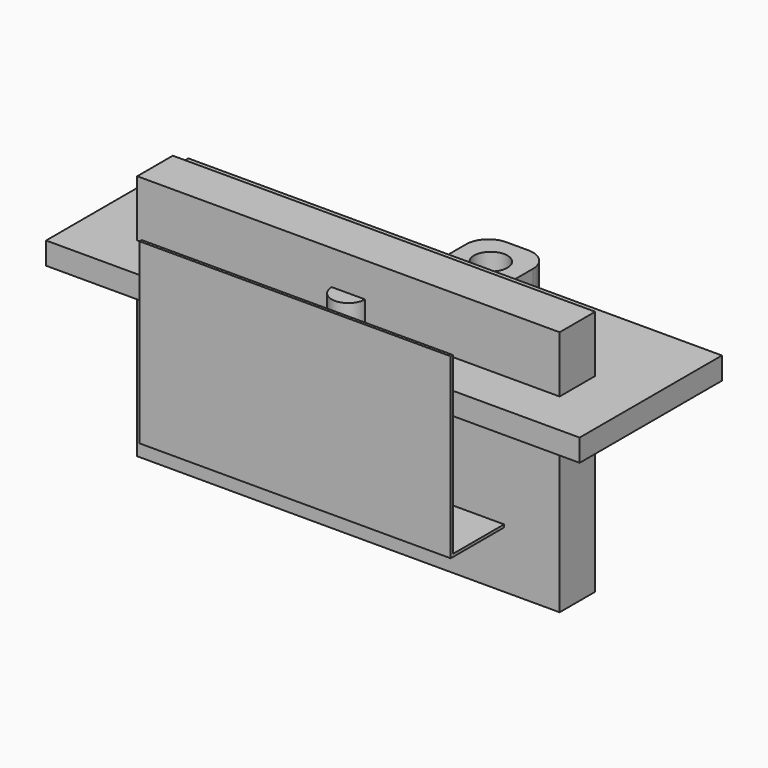
from build123d import *

# Parameters (mm, degrees)
F0_R           = 25.4
F1_DEPTH       = 50.8
F2_R           = 19.05
F3_DEPTH       = 50.8
F4_W           = 76.2
F4_H           = 254
F4_R           = 19.05
F5_DEPTH       = 50.8
F6_R           = 19.05
F7_DEPTH       = 50.8
F8_R           = 25.4
F9_R           = 38.1
F9_R_2         = 19.05
F10_DEPTH      = 50.8
F11_W          = 609.6
F11_H          = 203.2
F12_DEPTH      = 25.4
F13_R          = 19.05
F14_DEPTH      = 50.8
F15_W          = 482.6
F15_H          = 281.6996272628
F16_DEPTH      = 50.8
F17_R          = 25.4
F18_DEPTH      = 50.8
F20_DEPTH      = 177.8
F20_DEPTH_BACK = 177.8


with BuildPart() as f1:
    # F0 (on Top) → F1 (new body)
    with BuildSketch(Plane.XY):
        with BuildLine():
            ThreePointArc((-50.8, 0), (0, -50.8), (50.8, 0))
            ThreePointArc((50.8, 0), (0, 50.8), (-50.8, 0))
        make_face()
        Circle(F0_R, mode=Mode.SUBTRACT)
        with BuildLine():
            Line((50.8, -152.4), (50.8, 0))
            ThreePointArc((50.8, 0), (0, -50.8), (-50.8, 0))
            Line((-50.8, 0), (-50.8, -152.4))
            Line((-50.8, -152.4), (50.8, -152.4))
        make_face()
    extrude(amount=F1_DEPTH)

    # F2 (on face) → F3 (join)
    with BuildSketch(Plane.XY.offset(50.8)):
        with Locations((0, -114.3)):
            Circle(F2_R)
    extrude(amount=F3_DEPTH)


with BuildPart() as f5:
    # F4 (on Top) → F5 (new body)
    with BuildSketch(Plane.XY):
        Rectangle(F4_W, F4_H)
        with Locations((0, 88.9)):
            Circle(F4_R, mode=Mode.SUBTRACT)
    extrude(amount=F5_DEPTH)

    # F6 (on face) → F7 (join)
    with BuildSketch(Plane.XY.offset(50.8)):
        with Locations((0, -88.9)):
            Circle(F6_R)
    extrude(amount=F7_DEPTH)

    # F8
    f8_edges = [f5.edges().sort_by_distance(p)[0] for p in [
        (-38.1, -127, 25.4),
        (38.1, -127, 25.4),
        (38.1, 127, 25.4),
        (-38.1, 127, 25.4),
    ]]
    fillet(f8_edges, radius=F8_R)


with BuildPart() as f10:
    # F9 (on Top) → F10 (new body)
    with BuildSketch(Plane.XY):
        Circle(F9_R)
        Circle(F9_R_2, mode=Mode.SUBTRACT)
    extrude(amount=F10_DEPTH)

    # F11 (on face) → F12 (join)
    with BuildSketch(Plane.XY.offset(50.8)):
        with Locations((0, -63.5)):
            Rectangle(F11_W, F11_H)
    extrude(amount=F12_DEPTH)


with BuildPart() as f14:
    # F13 (on Top) → F14 (new body)
    with BuildSketch(Plane.XY):
        with BuildLine():
            ThreePointArc((-38.1, 0), (0, -38.1), (38.1, 0))
            ThreePointArc((38.1, 0), (0, 38.1), (-38.1, 0))
        make_face()
        Circle(F13_R, mode=Mode.SUBTRACT)
        with BuildLine():
            Line((38.1, -63.5), (38.1, 0))
            ThreePointArc((38.1, 0), (0, -38.1), (-38.1, 0))
            Line((-38.1, 0), (-38.1, -63.5))
            Line((-38.1, -63.5), (38.1, -63.5))
        make_face()
    extrude(amount=F14_DEPTH)

    # F15 (on face) → F16 (join)
    with BuildSketch(Plane.XZ.offset(63.5)):
        Rectangle(F15_W, F15_H)
    extrude(amount=F16_DEPTH)


with BuildPart() as f18:
    # F17 (on Top) → F18 (new body)
    with BuildSketch(Plane.XY):
        with BuildLine():
            ThreePointArc((-50.8, 0), (0, -50.8), (50.8, 0))
            ThreePointArc((50.8, 0), (0, 50.8), (-50.8, 0))
        make_face()
        Circle(F17_R, mode=Mode.SUBTRACT)
        with BuildLine():
            Line((50.8, -76.2), (50.8, 0))
            ThreePointArc((50.8, 0), (0, -50.8), (-50.8, 0))
            Line((-50.8, 0), (-50.8, -76.2))
            Line((-50.8, -76.2), (50.8, -76.2))
        make_face()
    extrude(amount=F18_DEPTH)

    # F19 (on Right) → F20 (join, two sides)
    with BuildSketch(Plane.YZ) as f20_sk:
        Polygon((-76.2, 0), (-76.2, 50.8), (-76.2, 127), (-79.375, 127), (-79.375, -73.025), (-187.325, -73.025), (-187.325, 127), (-190.5, 127), (-190.5, -76.2), (-76.2, -76.2), align=None)
    extrude(amount=F20_DEPTH)
    extrude(f20_sk.sketch, amount=-F20_DEPTH_BACK)


solid = Compound([f1.part, f5.part, f10.part, f14.part, f18.part])
